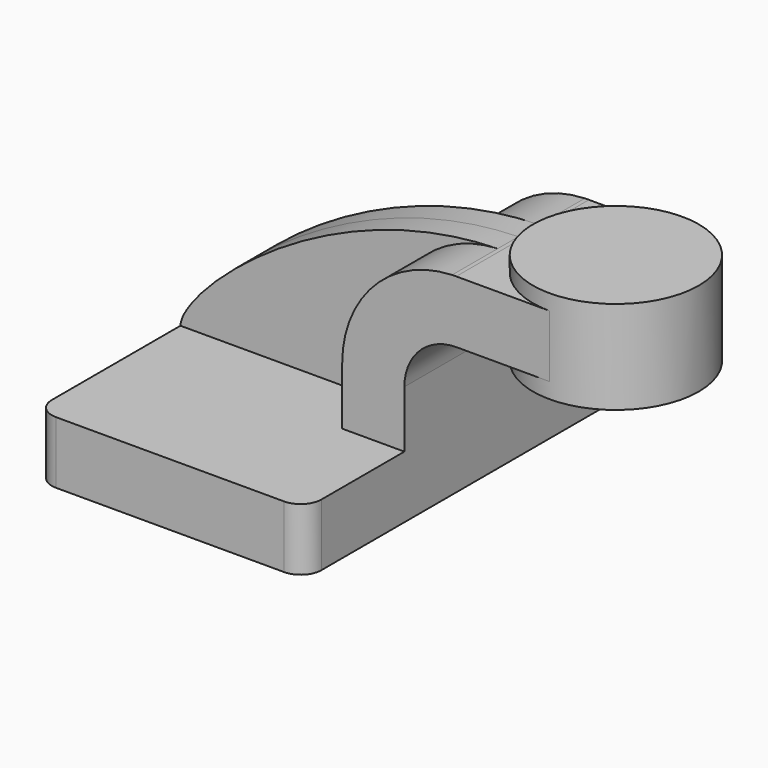
from build123d import *

# Parameters (mm, degrees)
F1_DEPTH = 25
F0_W     = 10
F0_H     = 7.5
F2_DEPTH = 10
F3_DEPTH = 3.125
F5_R     = 2.5


# Not quite as in the source:
# - a feature names something its author has since deleted; it is built from what else it names


with BuildPart() as f1:
    # F0 (on Front) → F1 (new body, symmetric)
    with BuildSketch(Plane.XZ):
        Polygon((16.25, -3.75), (16.25, 3.75), (8.75, 3.75), (-16.25, 3.75), (-16.25, -3.75), align=None)
    extrude(amount=F1_DEPTH, both=True)

    # F0 (on Front) → F2 (join, symmetric)
    with BuildSketch(Plane.XZ):
        with BuildLine():
            Line((8.75, 3.75), (16.25, 3.75))
            Line((16.25, 3.75), (16.25, 10.63))
            ThreePointArc((16.25, 10.63), (18.0805826176, 15.0494173824), (22.5, 16.88))
            Line((22.5, 16.88), (23.75, 16.88))
            Line((23.75, 16.88), (23.75, 24.38))
            Line((23.75, 24.38), (22.5, 24.38))
            add(Edge.make_bspline(
                [(22.0015189443, 24.3709612705), (22.1674265419, 24.3749356352), (22.3335889493, 24.3779529773), (22.5, 24.38)],
                knots=[43.5574597922, 43.5574597922, 43.5574597922, 43.5574597922, 43.8994236864, 43.8994236864, 43.8994236864, 43.8994236864], degree=3))
            ThreePointArc((22.0015189443, 24.3709612705), (12.6026110889, 20.1748516354), (8.75, 10.63))
            Line((8.75, 10.63), (8.75, 3.75))
        make_face()
        with Locations((28.75, 20.63)):
            Rectangle(F0_W, F0_H)
    extrude(amount=F2_DEPTH, both=True)

    # F0 (on Front) → F3 (join, symmetric)
    with BuildSketch(Plane.XZ):
        with BuildLine():
            Line((-16.25, 3.75), (8.75, 3.75))
            Line((8.75, 3.75), (8.75, 10.63))
            ThreePointArc((8.75, 10.63), (12.6026110889, 20.1748516354), (22.0015189443, 24.3709612705))
            add(Edge.make_bspline(
                [(-16.25, 3.75), (-16.1291590572, 7.8315246284), (0.86913148, 23.864728791), (22.0015189443, 24.3709612705)],
                knots=[0, 0, 0, 0, 43.5574597922, 43.5574597922, 43.5574597922, 43.5574597922], degree=3))
        make_face()
    extrude(amount=F3_DEPTH, both=True)

    # F0 (on Front) → F4 (revolve)
    with BuildSketch(Plane.XZ):
        Polygon((33.75, 24.38), (33.75, 16.88), (33.75, 15), (43.75, 15), (43.75, 26.25), (33.75, 26.25), align=None)
    revolve(axis=Axis((33.75, 0, 20.625), (0, 0, -1)))

    # F5
    f5_edges = [f1.edges().sort_by_distance(p)[0] for p in [
        (-16.25, -25, 0),
        (16.25, -25, 0),
        (-16.25, 25, 0),
        (16.25, 25, 0),
    ]]
    fillet(f5_edges, radius=F5_R)


solid = f1.part
